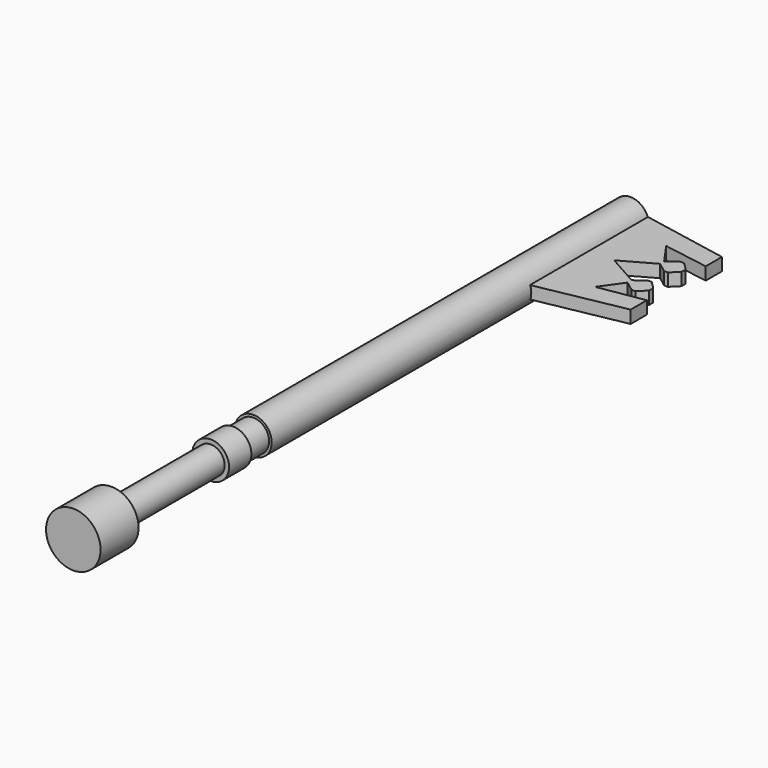
from build123d import *

# Parameters (mm, degrees)
F0_R      = 29
F1_DEPTH  = 750
F2_R      = 25
F3_DEPTH  = 40
F4_R      = 29
F4_R_2    = 25
F5_DEPTH  = 44
F6_R      = 22
F7_DEPTH  = 196
F8_R      = 43
F8_R_2    = 22
F9_DEPTH  = 75
F10_SIZE2 = 25
F10_SIZE  = 6
F11_W     = 6
F11_H     = 12
F12_DEPTH = 10


# Not quite as in the source:
# - a feature names something its author has since deleted; it is built from what else it names


with BuildPart() as f1:
    # F0 (on Front) → F1 (new body)
    with BuildSketch(Plane.XZ):
        Circle(F0_R)
    extrude(amount=-F1_DEPTH)

    # F2 (on Front) → F3 (join)
    with BuildSketch(Plane.XZ):
        Circle(F2_R)
    extrude(amount=F3_DEPTH)

    # F4 (on face) → F5 (join)
    with BuildSketch(Plane.XZ.offset(40)):
        Circle(F4_R)
        Circle(F4_R_2, mode=Mode.SUBTRACT)
        Circle(F4_R_2)
    extrude(amount=F5_DEPTH)

    # F6 (on face) → F7 (join)
    with BuildSketch(Plane.XZ.offset(84)):
        Circle(F6_R)
    extrude(amount=F7_DEPTH)

    # F8 (on face) → F9 (join)
    with BuildSketch(Plane.XZ.offset(280)):
        Circle(F8_R)
        Circle(F8_R_2, mode=Mode.SUBTRACT)
        Circle(F8_R_2)
    extrude(amount=F9_DEPTH)

    # F10
    f10_edges = [f1.edges().sort_by_distance(p)[0] for p in [
        (-29, 750, 0),
    ]]
    f10_side = f1.faces().sort_by_distance((-29, 375, 0))[0]
    chamfer(f10_edges, length=F10_SIZE, length2=F10_SIZE2, reference=f10_side)

    # F11 (on Top) → F12 (join, symmetric)
    with BuildSketch(Plane.XY):
        Polygon((164.9999544621, 717.9999580383), (28.9999544621, 743.9999580383), (28.9999544621, 717.9999580383), align=None)
        Polygon((28.9999544621, 717.9999580383), (28.9999544621, 743.9999580383), (3.9999544621, 743.9999580383), (3.9999544621, 511.9999580383), (28.9999544621, 511.9999580383), (28.9999544621, 537.9999580383), align=None)
        Polygon((164.9999544621, 717.9999580383), (28.9999544621, 717.9999580383), (28.9999544621, 537.9999580383), (164.9999544621, 537.9999580383), (164.9999544621, 557.9999580383), (92.9999544621, 557.9999580383), (92.9999544621, 591.9999580383), (66.9999544621, 591.9999580383), (66.9999544621, 599.9999580383), (66.9999544621, 627.9999580383), (66.9999544621, 655.9999580383), (92.9999544621, 655.9999580383), (92.9999544621, 663.9999580383), (92.9999544621, 697.9999580383), (164.9999544621, 697.9999580383), align=None)
        Polygon((164.9999544621, 537.9999580383), (28.9999544621, 537.9999580383), (28.9999544621, 511.9999580383), align=None)
        Polygon((164.9999544621, 685.9999580383), (164.9999544621, 697.9999580383), (92.9999544621, 697.9999580383), align=None)
        Polygon((116.9999544621, 663.9999580383), (92.9999544621, 697.9999580383), (92.9999544621, 663.9999580383), align=None)
        Polygon((92.9999544621, 557.9999580383), (164.9999544621, 557.9999580383), (164.9999544621, 569.9999580383), align=None)
        Polygon((116.9999544621, 663.9999580383), (92.9999544621, 663.9999580383), (92.9999544621, 655.9999580383), (116.9999544621, 655.9999580383), (132.9999544621, 655.9999580383), (138.9999544621, 655.9999580383), (150.9999544621, 655.9999580383), (150.9999544621, 663.9999580383), (138.9999544621, 663.9999580383), (132.9999544621, 663.9999580383), align=None)
        Polygon((132.9999544621, 675.9999580383), (116.9999544621, 663.9999580383), (132.9999544621, 663.9999580383), align=None)
        Polygon((92.9999544621, 591.9999580383), (92.9999544621, 557.9999580383), (116.9999544621, 591.9999580383), align=None)
        Polygon((116.9999544621, 655.9999580383), (92.9999544621, 655.9999580383), (66.9999544621, 655.9999580383), (66.9999544621, 627.9999580383), align=None)
        with Locations((135.9999544621, 669.9999580383)):
            Rectangle(F11_W, F11_H)
        Polygon((66.9999544621, 591.9999580383), (92.9999544621, 591.9999580383), (116.9999544621, 591.9999580383), (132.9999544621, 591.9999580383), (138.9999544621, 591.9999580383), (150.9999544621, 591.9999580383), (150.9999544621, 599.9999580383), (138.9999544621, 599.9999580383), (132.9999544621, 599.9999580383), (116.9999544621, 599.9999580383), (66.9999544621, 599.9999580383), align=None)
        Polygon((132.9999544621, 591.9999580383), (116.9999544621, 591.9999580383), (132.9999544621, 579.9999580383), align=None)
        Polygon((132.9999544621, 655.9999580383), (116.9999544621, 655.9999580383), (132.9999544621, 643.9999580383), align=None)
        Polygon((138.9999544621, 675.9999580383), (138.9999544621, 663.9999580383), (150.9999544621, 663.9999580383), align=None)
        with Locations((135.9999544621, 585.9999580383)):
            Rectangle(F11_W, F11_H)
        with Locations((135.9999544621, 649.9999580383)):
            Rectangle(F11_W, F11_H)
        Polygon((116.9999544621, 599.9999580383), (66.9999544621, 627.9999580383), (66.9999544621, 599.9999580383), align=None)
        Polygon((150.9999544621, 591.9999580383), (138.9999544621, 591.9999580383), (138.9999544621, 579.9999580383), align=None)
        Polygon((150.9999544621, 655.9999580383), (138.9999544621, 655.9999580383), (138.9999544621, 643.9999580383), align=None)
        Polygon((132.9999544621, 611.9999580383), (116.9999544621, 599.9999580383), (132.9999544621, 599.9999580383), align=None)
        with Locations((135.9999544621, 605.9999580383)):
            Rectangle(F11_W, F11_H)
        Polygon((138.9999544621, 599.9999580383), (150.9999544621, 599.9999580383), (138.9999544621, 611.9999580383), align=None)
    extrude(amount=F12_DEPTH, both=True)


solid = f1.part
